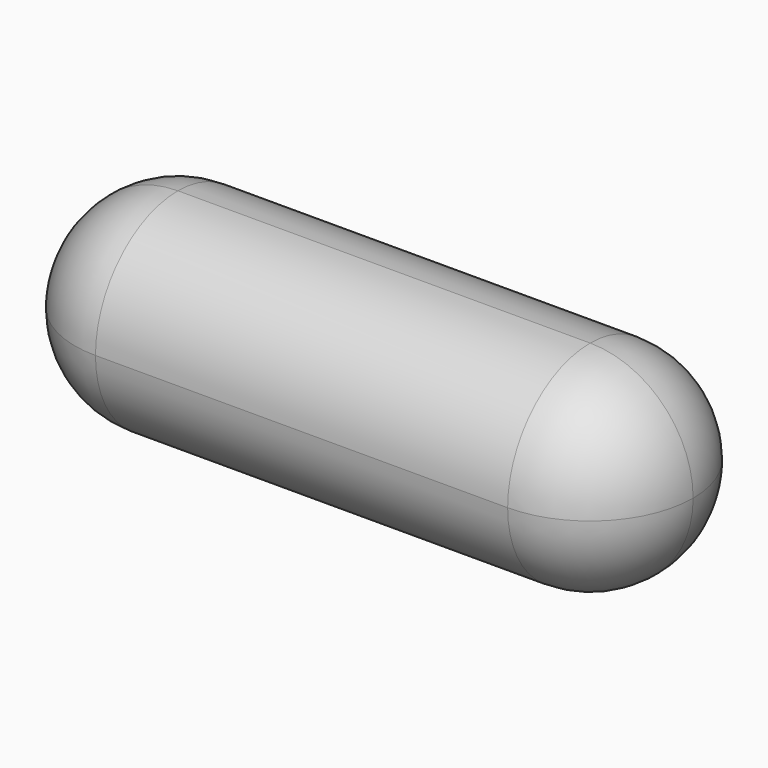
from build123d import *

# Parameters (mm, degrees)
F0_W     = 30
F0_H     = 10
F1_DEPTH = 10
F2_R     = 4.99999
F3_R     = 4.99999


# Not quite as in the source:
# - a fillet or chamfer is up to 0.001 mm smaller than in the source, because OpenCascade refuses the exact size


with BuildPart() as f1:
    # F0 (on Top) → F1 (new body)
    with BuildSketch(Plane.XY):
        with Locations((15, 5)):
            Rectangle(F0_W, F0_H)
    extrude(amount=F1_DEPTH)

    # F2 (radius 5 in the source; OpenCascade refuses exactly that, so slightly less here)
    f2_edges = [f1.edges().sort_by_distance(p)[0] for p in [
        (15, 0, 10),
        (15, 0, 0),
        (15, 10, 0),
        (15, 10, 10),
    ]]
    fillet(f2_edges, radius=F2_R)

    # F3 (radius 5 in the source; OpenCascade refuses exactly that, so slightly less here)
    f3_edges = [f1.edges().sort_by_distance(p)[0] for p in [
        (30, 0, 5),
        (30, 1.464463, 1.464463),
        (30, 1.464463, 8.535537),
        (30, 5, 0),
        (30, 5, 10),
        (30, 8.535537, 1.464463),
        (30, 8.535537, 8.535537),
        (30, 10, 5),
        (0, 10, 5),
        (0, 8.535537, 1.464463),
        (0, 8.535537, 8.535537),
        (0, 5, 0),
        (0, 5, 10),
        (0, 1.464463, 1.464463),
        (0, 1.464463, 8.535537),
        (0, 0, 5),
    ]]
    fillet(f3_edges, radius=F3_R)


solid = f1.part
